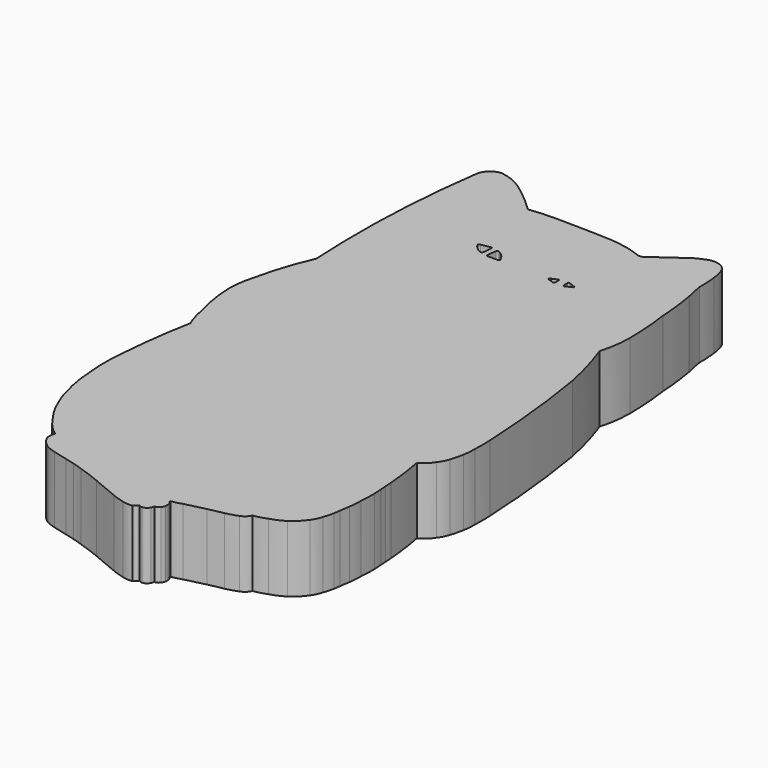
from build123d import *

# Parameters (mm, degrees)
F0_R     = 0.4870589974
F0_R_2   = 0.3474724492
F0_R_3   = 0.3665024193
F0_R_4   = 0.3542305884
F2_DEPTH = 15.24


# Not quite as in the source:
# - the program builds the solid bodies; features that only make, move or delete a surface that nothing else refers to are left out


with BuildPart() as f2:
    # F0 (on Top) → F2 (new body)
    with BuildSketch(Plane.XY):
        with BuildLine():
            ThreePointArc((-4.6574980952, 64.4998699427), (-8.9647320566, 64.5008636046), (-13.2575705647, 64.1490072012))
            ThreePointArc((-13.2575705647, 64.1490072012), (-16.5825370368, 67.1811284014), (-20.1327186078, 69.946154952))
            ThreePointArc((-20.1327186078, 69.946154952), (-22.7316970175, 71.3928848027), (-25.5997013301, 72.1817240119))
            ThreePointArc((-25.5997013301, 72.1817240119), (-27.9785809795, 71.1960010823), (-29.0786921978, 68.8678100705))
            ThreePointArc((-29.0786921978, 68.8678100705), (-31.0430656712, 47.2705474966), (-30.8605283499, 25.5849026144))
            ThreePointArc((-30.8605283499, 25.5849026144), (-33.274027732, 19.3250082515), (-35.0082106888, 12.843969278))
            ThreePointArc((-35.0082106888, 12.843969278), (-35.6586909212, 9.8700411989), (-35.8947664499, 6.8349726498))
            ThreePointArc((-35.8947664499, 6.8349726498), (-35.4181204016, 1.9087445697), (-34.3186743557, -2.9168261681))
            ThreePointArc((-34.3186743557, -2.9168261681), (-33.7425928924, -5.5247875256), (-32.8410901129, -8.0388728529))
            ThreePointArc((-32.8410901129, -8.0388728529), (-34.177182437, -16.2583737842), (-35.0319556892, -24.541772902))
            ThreePointArc((-35.0319556892, -24.541772902), (-35.3040614644, -29.3553117663), (-35.0319556892, -34.1688506305))
            ThreePointArc((-35.0319556892, -34.1688506305), (-34.5298956541, -38.6068361214), (-33.4818251431, -42.9484173656))
            ThreePointArc((-33.4818251431, -42.9484173656), (-33.0135473697, -44.5160756792), (-32.4171707034, -46.0396148264))
            ThreePointArc((-32.4171707034, -46.0396148264), (-31.9110692256, -47.2219894678), (-31.3906520605, -48.3981333673))
            ThreePointArc((-31.3906520605, -48.3981333673), (-30.5934071364, -49.8697175037), (-29.6822413802, -51.2736178935))
            ThreePointArc((-29.6822413802, -51.2736178935), (-28.7221089025, -52.6566027976), (-27.7248732746, -54.0130771697))
            ThreePointArc((-27.7248732746, -54.0130771697), (-26.4672846913, -55.3801105964), (-25.0454377383, -56.5753765404))
            Line((-25.0454377383, -56.5753765404), (-24.942945689, -56.6339418292))
            ThreePointArc((-24.942945689, -56.6339418292), (-25.1177355033, -57.0589329105), (-25.1918546855, -57.512447238))
            ThreePointArc((-25.1918546855, -57.512447238), (-25.1982887044, -58.3404447624), (-24.9355826527, -59.125687927))
            ThreePointArc((-24.9355826527, -59.125687927), (-24.0502846613, -60.3263263494), (-22.9040738195, -61.2810440361))
            ThreePointArc((-22.9040738195, -61.2810440361), (-21.8272966835, -61.7764366965), (-20.7001958042, -62.1431879699))
            ThreePointArc((-20.7001958042, -62.1431879699), (-19.0633016555, -62.5643833918), (-17.4251589924, -62.980696559))
            ThreePointArc((-17.4251589924, -62.980696559), (-16.3259212101, -63.2570568454), (-15.2335911989, -63.5595694184))
            ThreePointArc((-15.2335911989, -63.5595694184), (-14.0547489271, -63.8999797911), (-12.8942783922, -64.2985478044))
            ThreePointArc((-12.8942783922, -64.2985478044), (-10.3776553028, -65.1515690841), (-7.898459211, -66.1079287529))
            ThreePointArc((-7.898459211, -66.1079287529), (-4.843659707, -67.400231929), (-1.7793092411, -68.6697214842))
            ThreePointArc((-1.7793092411, -68.6697214842), (-0.4258068603, -69.1536416461), (0.953993469, -69.556504488))
            ThreePointArc((0.953993469, -69.556504488), (2.09089533, -69.7563797595), (3.2440575305, -69.7042942047))
            ThreePointArc((3.2440575305, -69.7042942047), (3.7517072509, -69.2953475436), (4.1341194883, -68.7674209476))
            ThreePointArc((4.1341194883, -68.7674209476), (4.4824361357, -69.0112523604), (4.9028098583, -69.0750032663))
            ThreePointArc((4.9028098583, -69.0750032663), (5.6978837565, -68.8446948411), (6.2388665974, -68.2181790471))
            ThreePointArc((6.2388665974, -68.2181790471), (6.3961650377, -67.8668892643), (6.4935988233, -67.4945265805))
            ThreePointArc((6.4935988233, -67.4945265805), (7.0853776684, -67.3748926573), (7.5344089419, -66.9713020325))
            ThreePointArc((7.5344089419, -66.9713020325), (7.7893950341, -66.5594064291), (7.9566510394, -66.1047622561))
            ThreePointArc((7.9566510394, -66.1047622561), (7.9580850948, -65.3933472028), (7.7242949046, -64.721442759))
            ThreePointArc((7.7242949046, -64.721442759), (7.6240357038, -64.5454642025), (7.4602863751, -64.4262731075))
            Line((7.4602863751, -64.4262731075), (7.4602863751, -64.1000345349))
            ThreePointArc((7.4602863751, -64.1000345349), (8.6957807292, -63.8684813987), (9.8980711773, -63.5016560555))
            ThreePointArc((9.8980711773, -63.5016560555), (12.1765605556, -62.956644983), (14.4535750151, -62.4055042863))
            ThreePointArc((14.4535750151, -62.4055042863), (16.1980956729, -62.0296921019), (17.9502312094, -61.6911537945))
            ThreePointArc((17.9502312094, -61.6911537945), (19.3508412218, -61.3167352774), (20.720468834, -60.8413219452))
            ThreePointArc((20.720468834, -60.8413219452), (21.7172842906, -60.2151089758), (22.3949253559, -59.2525154352))
            ThreePointArc((22.3949253559, -59.2525154352), (23.9413170616, -58.9427415638), (25.4360325634, -58.4396384656))
            ThreePointArc((25.4360325634, -58.4396384656), (27.0823885834, -57.8282787188), (28.6495089531, -57.0355728269))
            ThreePointArc((28.6495089531, -57.0355728269), (30.1858910448, -55.7262813708), (31.481307, -54.1781820357))
            ThreePointArc((31.481307, -54.1781820357), (32.1372272216, -53.052991053), (32.5707420707, -51.8248416483))
            ThreePointArc((32.5707420707, -51.8248416483), (32.9555178669, -50.6466711835), (33.2324020565, -49.4385845959))
            ThreePointArc((33.2324020565, -49.4385845959), (33.3537864539, -48.7541435906), (33.4239304066, -48.0625703931))
            ThreePointArc((33.4239304066, -48.0625703931), (33.5955437011, -46.9075690976), (33.7808765471, -45.7546897233))
            ThreePointArc((33.7808765471, -45.7546897233), (33.9514589063, -44.2393966213), (33.9985303581, -42.7152588964))
            ThreePointArc((33.9985303581, -42.7152588964), (34.1163088336, -40.8315734776), (34.118514508, -38.9442108572))
            ThreePointArc((34.118514508, -38.9442108572), (34.083978003, -37.9792527189), (33.9942798018, -37.0178520679))
            ThreePointArc((33.9942798018, -37.0178520679), (33.955975515, -36.2784612284), (33.8882356882, -35.5411842465))
            ThreePointArc((33.8882356882, -35.5411842465), (33.8712782201, -34.6642287786), (33.786136657, -33.7912514806))
            ThreePointArc((33.786136657, -33.7912514806), (33.3180795223, -29.3661557271), (32.5943753123, -24.9756202102))
            ThreePointArc((32.5943753123, -24.9756202102), (34.0489107492, -23.9527476363), (35.1713187993, -22.5735660642))
            ThreePointArc((35.1713187993, -22.5735660642), (35.9010770472, -21.4620836312), (36.4012233913, -20.2300958335))
            ThreePointArc((36.4012233913, -20.2300958335), (36.828967703, -18.7660485621), (37.1333099902, -17.2714665532))
            ThreePointArc((37.1333099902, -17.2714665532), (37.3389003532, -15.7697261697), (37.3675785959, -14.2542496324))
            ThreePointArc((37.3675785959, -14.2542496324), (37.4263640724, -12.1011873707), (37.3675785959, -9.9481251091))
            ThreePointArc((37.3675785959, -9.9481251091), (36.331409459, 3.6788193791), (34.4893857837, 17.2203928232))
            ThreePointArc((34.4893857837, 17.2203928232), (33.0120348597, 23.3170518073), (31.0925077647, 29.2892567813))
            ThreePointArc((31.0925077647, 29.2892567813), (31.8892450574, 32.9417140758), (32.1467109025, 36.6711840034))
            ThreePointArc((32.1467109025, 36.6711840034), (31.9281916192, 41.8984630944), (31.3738137484, 47.1008531749))
            ThreePointArc((31.3738137484, 47.1008531749), (30.9870656208, 51.5076967811), (30.3440932184, 55.8845028281))
            ThreePointArc((30.3440932184, 55.8845028281), (29.8980506559, 57.8596492724), (29.5387990773, 59.8524101079))
            ThreePointArc((29.5387990773, 59.8524101079), (29.5001644092, 62.03824233), (29.3045323342, 64.2156451941))
            ThreePointArc((29.3045323342, 64.2156451941), (29.0554228466, 65.8357987344), (28.5431630909, 67.3928931355))
            ThreePointArc((28.5431630909, 67.3928931355), (27.7313873665, 68.4152918791), (26.5811719, 69.0327733755))
            ThreePointArc((26.5811719, 69.0327733755), (25.4317978397, 69.2090389422), (24.2824237794, 69.0327733755))
            ThreePointArc((24.2824237794, 69.0327733755), (21.9444120738, 68.0189193625), (19.8459811509, 66.5729641914))
            ThreePointArc((19.8459811509, 66.5729641914), (17.3300117141, 64.7862316617), (14.8238698021, 62.985740602))
            ThreePointArc((14.8238698021, 62.985740602), (14.2064215735, 62.5788950359), (13.4768299758, 62.4586381018))
            ThreePointArc((13.4768299758, 62.4586381018), (11.0316395646, 63.3169292546), (8.4986444563, 63.8642460108))
            ThreePointArc((8.4986444563, 63.8642460108), (6.8510393358, 64.1197437557), (5.1896148361, 64.2595663667))
            ThreePointArc((5.1896148361, 64.2595663667), (0.2670117865, 64.4187870504), (-4.6574980952, 64.4998699427))
        make_face()
        with BuildLine():
            Line((-1.0718253907, -67.4767941236), (6.3647264615, -64.5711272955))
            ThreePointArc((6.3647264615, -64.5711272955), (6.9733703953, -65.3588843298), (6.8818381988, -66.3501615061))
            ThreePointArc((6.8818381988, -66.3501615061), (6.248455993, -66.5475154041), (5.7491185144, -66.9843032956))
            ThreePointArc((5.7491185144, -66.9843032956), (5.5498506128, -67.2328710451), (5.5274991319, -67.5506666303))
            ThreePointArc((5.5274991319, -67.5506666303), (5.4100983825, -67.8395088195), (5.1088854671, -67.9200291634))
            ThreePointArc((5.1088854671, -67.9200291634), (4.550994403, -67.8804673339), (4.0992875583, -67.5506666303))
            ThreePointArc((4.0992875583, -67.5506666303), (3.689928496, -67.5720046833), (3.3851813059, -67.8461566567))
            ThreePointArc((3.3851813059, -67.8461566567), (3.1917592991, -68.325763414), (2.8434458654, -68.7080100179))
            ThreePointArc((2.8434458654, -68.7080100179), (2.3263345356, -68.8067226844), (1.8092232058, -68.7080100179))
            ThreePointArc((1.8092232058, -68.7080100179), (0.3713994895, -68.2197332578), (-1.0718253907, -67.7476599813))
            ThreePointArc((-1.0718253907, -67.7476599813), (-1.1643120138, -67.6122270525), (-1.0718253907, -67.4767941236))
        make_face(mode=Mode.SUBTRACT)
        with BuildLine():
            ThreePointArc((-2.623158507, -65.6792148948), (-2.6954743039, -64.9004723873), (-2.5739099365, -64.1278848052))
            ThreePointArc((-2.5739099365, -64.1278848052), (-2.7480826507, -63.9151836223), (-3.017146606, -63.858769834))
            ThreePointArc((-3.017146606, -63.858769834), (-3.4181090068, -63.7899955014), (-3.7558770273, -63.5632500052))
            ThreePointArc((-3.7558770273, -63.5632500052), (-4.1021139481, -62.8983397037), (-3.7558770273, -62.2334294021))
            ThreePointArc((-3.7558770273, -62.2334294021), (-3.4445311977, -61.8172751284), (-3.4357607365, -61.2976178527))
            ThreePointArc((-3.4357607365, -61.2976178527), (-3.8185334208, -61.0520831854), (-4.2483638972, -60.9035976231))
            ThreePointArc((-4.2483638972, -60.9035976231), (-4.256998038, -60.2746639674), (-4.0759937838, -59.6722774208))
            ThreePointArc((-4.0759937838, -59.6722774208), (-2.988790696, -58.6144122793), (-1.6381832538, -57.923797518))
            ThreePointArc((-1.6381832538, -57.923797518), (1.1811274388, -56.897382154), (3.9022939745, -55.6335411966))
            ThreePointArc((3.9022939745, -55.6335411966), (5.981824211, -53.9429218927), (7.5466968119, -51.7671890557))
            ThreePointArc((7.5466968119, -51.7671890557), (8.3550122972, -52.4735297418), (9.368898347, -52.8261289001))
            ThreePointArc((9.368898347, -52.8261289001), (10.040849572, -52.6552470488), (9.9845072255, -51.9642010331))
            ThreePointArc((9.9845072255, -51.9642010331), (8.9657442091, -51.4896380021), (8.1130573526, -50.7575087249))
            ThreePointArc((8.1130573526, -50.7575087249), (7.7223088512, -49.166699086), (7.4235755019, -47.5560724735))
            ThreePointArc((7.4235755019, -47.5560724735), (7.2790449544, -44.2315042019), (7.4235755019, -40.9069359303))
            ThreePointArc((7.4235755019, -40.9069359303), (7.8475833512, -38.1104558628), (8.5316719487, -35.3659875691))
            ThreePointArc((8.5316719487, -35.3659875691), (9.546237916, -32.4876606134), (10.8463596553, -29.7265388072))
            ThreePointArc((10.8463596553, -29.7265388072), (12.7163248023, -26.7781756457), (15.0817465037, -24.2102202028))
            ThreePointArc((15.0817465037, -24.2102202028), (18.4017864047, -21.252419583), (22.2720559686, -19.0632957965))
            ThreePointArc((22.2720559686, -19.0632957965), (23.6866847639, -20.4435503048), (25.0792298466, -21.8460820615))
            ThreePointArc((25.0792298466, -21.8460820615), (28.1924648647, -24.0565281675), (31.6785536706, -25.6139263511))
            ThreePointArc((31.6785536706, -25.6139263511), (32.1205537257, -27.5065827192), (32.3926620185, -29.4310227036))
            ThreePointArc((32.3926620185, -29.4310227036), (32.7406981771, -31.9726512024), (32.9590179026, -34.5286913216))
            ThreePointArc((32.9590179026, -34.5286913216), (33.1425338772, -37.1117354068), (33.2052633166, -39.7005304694))
            ThreePointArc((33.2052633166, -39.7005304694), (33.1792019702, -43.1222482344), (32.7866487205, -46.521473676))
            ThreePointArc((32.7866487205, -46.521473676), (32.2374801563, -49.6606541109), (31.2106925994, -52.6775643229))
            ThreePointArc((31.2106925994, -52.6775643229), (29.6463762239, -54.7894621513), (27.5662895292, -56.3958361745))
            ThreePointArc((27.5662895292, -56.3958361745), (25.1040574774, -57.5429066445), (22.4444251508, -58.0949150026))
            ThreePointArc((22.4444251508, -58.0949150026), (22.1710291401, -57.487026745), (21.8780655414, -56.8883232772))
            ThreePointArc((21.8780655414, -56.8883232772), (21.2040875244, -56.5900957809), (20.8438429981, -57.2330653667))
            ThreePointArc((20.8438429981, -57.2330653667), (21.2474215961, -58.0165612606), (21.5086974204, -58.8582716882))
            ThreePointArc((21.5086974204, -58.8582716882), (20.6940197818, -59.6369824276), (19.661873579, -60.0894913077))
            Line((19.661873579, -60.0894913077), (7.3989494704, -63.0690380931))
            Line((7.3989494704, -63.0690380931), (2.3263345938, -64.7681206465))
            ThreePointArc((2.3263345938, -64.7681206465), (0.5926919978, -65.3977667437), (-1.0189079934, -66.2948265672))
            ThreePointArc((-1.0189079934, -66.2948265672), (-1.9152742777, -66.2326077196), (-2.623158507, -65.6792148948))
        make_face(mode=Mode.SUBTRACT)
        with Locations((-6.3439328223, 36.2661853433)):
            Circle(F0_R, mode=Mode.SUBTRACT)
        with Locations((-4.6601346694, 35.225212574)):
            Circle(F0_R_2, mode=Mode.SUBTRACT)
        with BuildLine():
            ThreePointArc((-24.7670784593, 67.2100633383), (-24.7422360081, 67.4660931138), (-24.5035272092, 67.5619393587))
            ThreePointArc((-24.5035272092, 67.5619393587), (-24.2630023675, 67.5067616438), (-24.0935590118, 67.3273578286))
            Line((-24.0935590118, 67.3273578286), (-20.2720686793, 63.7499317527))
            ThreePointArc((-20.2720686793, 63.7499317527), (-20.1529238407, 63.5519680773), (-20.1110094786, 63.3247494698))
            ThreePointArc((-20.1110094786, 63.3247494698), (-20.1793091244, 63.1254039906), (-20.3599203378, 63.0168542266))
            Line((-20.3599203378, 63.0168542266), (-23.2150536031, 61.3798877609))
            ThreePointArc((-23.2150536031, 61.3798877609), (-23.4814881607, 61.1666838735), (-23.8153655082, 61.0961914062))
            ThreePointArc((-23.8153655082, 61.0961914062), (-24.0717534356, 61.1512212134), (-24.1814088076, 61.3894201815))
            Line((-24.1814088076, 61.3894201815), (-24.7670784593, 67.2100633383))
        make_face(mode=Mode.SUBTRACT)
        with BuildLine():
            ThreePointArc((-9.2142317444, 48.5497191548), (-8.9722191607, 48.5070335326), (-8.8777504861, 48.2801683247))
            Line((-8.8777504861, 48.2801683247), (-9.1055221856, 46.1445078254))
            ThreePointArc((-9.1055221856, 46.1445078254), (-9.450986085, 45.9388162481), (-9.84578114, 46.0149161518))
            ThreePointArc((-9.84578114, 46.0149161518), (-10.8691429713, 46.7574912238), (-11.6886617616, 47.7203391492))
            ThreePointArc((-11.6886617616, 47.7203391492), (-11.6248552564, 48.0182618453), (-11.3677093759, 48.1816790998))
            Line((-11.3677093759, 48.1816790998), (-9.2142317444, 48.5497191548))
        make_face(mode=Mode.SUBTRACT)
        with BuildLine():
            ThreePointArc((0.0798076726, 36.0665917397), (-0.924263096, 37.2791040663), (-1.5656301985, 38.7168079615))
            ThreePointArc((-1.5656301985, 38.7168079615), (0.3771124535, 38.733779164), (2.2301948629, 38.1501503289))
            ThreePointArc((2.2301948629, 38.1501503289), (2.234031658, 38.0462048397), (2.1953706164, 37.9496403039))
            ThreePointArc((2.1953706164, 37.9496403039), (1.2064186028, 36.9307876648), (0.0798076726, 36.0665917397))
        make_face(mode=Mode.SUBTRACT)
        with BuildLine():
            ThreePointArc((-7.5725880452, 47.912247479), (-7.3780353415, 48.1541943288), (-7.067638915, 48.1476299465))
            ThreePointArc((-7.067638915, 48.1476299465), (-5.8641532243, 47.2968616284), (-5.030429922, 46.0815057158))
            ThreePointArc((-5.030429922, 46.0815057158), (-4.8961302642, 45.7175598685), (-5.1958444528, 45.4712584615))
            Line((-5.1958444528, 45.4712584615), (-7.4855275452, 45.4712584615))
            ThreePointArc((-7.4855275452, 45.4712584615), (-7.7517799665, 45.59444949), (-7.8685926273, 45.8635613322))
            Line((-7.8685926273, 45.8635613322), (-7.5725880452, 47.912247479))
        make_face(mode=Mode.SUBTRACT)
        with Locations((3.9052728098, 34.0376272798)):
            Circle(F0_R_3, mode=Mode.SUBTRACT)
        with Locations((6.3650822267, 34.961309284)):
            Circle(F0_R_4, mode=Mode.SUBTRACT)
        Polygon((5.4925759323, 45.4602651298), (8.4121963009, 46.7665418983), (8.5571417585, 44.3198606372), align=None, mode=Mode.SUBTRACT)
        Polygon((9.8616527393, 44.3198606372), (9.8616527393, 47.0153577626), (13.0711635575, 45.8542220294), align=None, mode=Mode.SUBTRACT)
        with BuildLine():
            ThreePointArc((19.9374128133, 59.918910265), (19.5176768801, 60.3374275402), (19.863538444, 60.8187951148))
            Line((19.863538444, 60.8187951148), (24.9115284532, 65.5284225941))
            ThreePointArc((24.9115284532, 65.5284225941), (25.740638025, 65.6767219123), (26.1427462101, 64.9366378784))
            Line((26.1427462101, 64.9366378784), (25.9457528591, 58.1311024725))
            ThreePointArc((25.9457528591, 58.1311024725), (25.9478496261, 57.8546128108), (25.6748851389, 57.8105524182))
            Line((25.6748851389, 57.8105524182), (19.9374128133, 59.918910265))
        make_face(mode=Mode.SUBTRACT)
        with BuildLine():
            ThreePointArc((-3.017146606, -63.858769834), (-2.7480826507, -63.9151836223), (-2.5739099365, -64.1278848052))
            ThreePointArc((-2.5739099365, -64.1278848052), (-2.6954743039, -64.9004723873), (-2.623158507, -65.6792148948))
            ThreePointArc((-2.623158507, -65.6792148948), (-1.9152742777, -66.2326077196), (-1.0189079934, -66.2948265672))
            ThreePointArc((-1.0189079934, -66.2948265672), (0.5926919978, -65.3977667437), (2.3263345938, -64.7681206465))
            Line((2.3263345938, -64.7681206465), (7.3989494704, -63.0690380931))
            Line((7.3989494704, -63.0690380931), (19.661873579, -60.0894913077))
            ThreePointArc((19.661873579, -60.0894913077), (20.6940197818, -59.6369824276), (21.5086974204, -58.8582716882))
            ThreePointArc((21.5086974204, -58.8582716882), (21.2474215961, -58.0165612606), (20.8438429981, -57.2330653667))
            ThreePointArc((20.8438429981, -57.2330653667), (21.2040875244, -56.5900957809), (21.8780655414, -56.8883232772))
            ThreePointArc((21.8780655414, -56.8883232772), (22.1710291401, -57.487026745), (22.4444251508, -58.0949150026))
            ThreePointArc((22.4444251508, -58.0949150026), (25.1040574774, -57.5429066445), (27.5662895292, -56.3958361745))
            ThreePointArc((27.5662895292, -56.3958361745), (29.6463762239, -54.7894621513), (31.2106925994, -52.6775643229))
            ThreePointArc((31.2106925994, -52.6775643229), (32.2374801563, -49.6606541109), (32.7866487205, -46.521473676))
            ThreePointArc((32.7866487205, -46.521473676), (33.1792019702, -43.1222482344), (33.2052633166, -39.7005304694))
            ThreePointArc((33.2052633166, -39.7005304694), (33.1425338772, -37.1117354068), (32.9590179026, -34.5286913216))
            ThreePointArc((32.9590179026, -34.5286913216), (32.7406981771, -31.9726512024), (32.3926620185, -29.4310227036))
            ThreePointArc((32.3926620185, -29.4310227036), (32.1205537257, -27.5065827192), (31.6785536706, -25.6139263511))
            ThreePointArc((31.6785536706, -25.6139263511), (28.1924648647, -24.0565281675), (25.0792298466, -21.8460820615))
            ThreePointArc((25.0792298466, -21.8460820615), (23.6866847639, -20.4435503048), (22.2720559686, -19.0632957965))
            ThreePointArc((22.2720559686, -19.0632957965), (18.4017864047, -21.252419583), (15.0817465037, -24.2102202028))
            ThreePointArc((15.0817465037, -24.2102202028), (12.7163248023, -26.7781756457), (10.8463596553, -29.7265388072))
            ThreePointArc((10.8463596553, -29.7265388072), (9.546237916, -32.4876606134), (8.5316719487, -35.3659875691))
            ThreePointArc((8.5316719487, -35.3659875691), (7.8475833512, -38.1104558628), (7.4235755019, -40.9069359303))
            ThreePointArc((7.4235755019, -40.9069359303), (7.2790449544, -44.2315042019), (7.4235755019, -47.5560724735))
            ThreePointArc((7.4235755019, -47.5560724735), (7.7223088512, -49.166699086), (8.1130573526, -50.7575087249))
            ThreePointArc((8.1130573526, -50.7575087249), (8.9657442091, -51.4896380021), (9.9845072255, -51.9642010331))
            ThreePointArc((9.9845072255, -51.9642010331), (10.040849572, -52.6552470488), (9.368898347, -52.8261289001))
            ThreePointArc((9.368898347, -52.8261289001), (8.3550122972, -52.4735297418), (7.5466968119, -51.7671890557))
            ThreePointArc((7.5466968119, -51.7671890557), (5.981824211, -53.9429218927), (3.9022939745, -55.6335411966))
            ThreePointArc((3.9022939745, -55.6335411966), (1.1811274388, -56.897382154), (-1.6381832538, -57.923797518))
            ThreePointArc((-1.6381832538, -57.923797518), (-2.988790696, -58.6144122793), (-4.0759937838, -59.6722774208))
            ThreePointArc((-4.0759937838, -59.6722774208), (-4.256998038, -60.2746639674), (-4.2483638972, -60.9035976231))
            ThreePointArc((-4.2483638972, -60.9035976231), (-3.8185334208, -61.0520831854), (-3.4357607365, -61.2976178527))
            ThreePointArc((-3.4357607365, -61.2976178527), (-3.4445311977, -61.8172751284), (-3.7558770273, -62.2334294021))
            ThreePointArc((-3.7558770273, -62.2334294021), (-4.1021139481, -62.8983397037), (-3.7558770273, -63.5632500052))
            ThreePointArc((-3.7558770273, -63.5632500052), (-3.4181090068, -63.7899955014), (-3.017146606, -63.858769834))
        make_face()
        with BuildLine():
            Line((24.9115284532, 65.5284225941), (19.863538444, 60.8187951148))
            ThreePointArc((19.863538444, 60.8187951148), (19.5176768801, 60.3374275402), (19.9374128133, 59.918910265))
            Line((19.9374128133, 59.918910265), (25.6748851389, 57.8105524182))
            ThreePointArc((25.6748851389, 57.8105524182), (25.9478496261, 57.8546128108), (25.9457528591, 58.1311024725))
            Line((25.9457528591, 58.1311024725), (26.1427462101, 64.9366378784))
            ThreePointArc((26.1427462101, 64.9366378784), (25.740638025, 65.6767219123), (24.9115284532, 65.5284225941))
        make_face()
        with BuildLine():
            Line((20.9922753274, 60.810495168), (24.698741734, 64.3975809216))
            ThreePointArc((24.698741734, 64.3975809216), (25.0690158468, 64.4878677154), (25.278525427, 64.1694962978))
            Line((25.278525427, 64.1694962978), (25.1128729433, 58.9858517051))
            ThreePointArc((25.1128729433, 58.9858517051), (24.8968366977, 58.6634817199), (24.5123840868, 58.7163046002))
            Line((24.5123840868, 58.7163046002), (20.9922753274, 59.918910265))
            ThreePointArc((20.9922753274, 59.918910265), (20.7188387044, 60.1168568588), (20.6032761511, 60.4340251692))
            Line((20.6032761511, 60.4340251692), (20.9922753274, 60.810495168))
        make_face(mode=Mode.SUBTRACT)
        with BuildLine():
            ThreePointArc((-24.0935590118, 67.3273578286), (-24.2630023675, 67.5067616438), (-24.5035272092, 67.5619393587))
            ThreePointArc((-24.5035272092, 67.5619393587), (-24.7422360081, 67.4660931138), (-24.7670784593, 67.2100633383))
            Line((-24.7670784593, 67.2100633383), (-24.1814088076, 61.3894201815))
            ThreePointArc((-24.1814088076, 61.3894201815), (-24.0717534356, 61.1512212134), (-23.8153655082, 61.0961914062))
            ThreePointArc((-23.8153655082, 61.0961914062), (-23.4814881607, 61.1666838735), (-23.2150536031, 61.3798877609))
            Line((-23.2150536031, 61.3798877609), (-20.3599203378, 63.0168542266))
            ThreePointArc((-20.3599203378, 63.0168542266), (-20.1793091244, 63.1254039906), (-20.1110094786, 63.3247494698))
            ThreePointArc((-20.1110094786, 63.3247494698), (-20.1529238407, 63.5519680773), (-20.2720686793, 63.7499317527))
            Line((-20.2720686793, 63.7499317527), (-24.0935590118, 67.3273578286))
        make_face()
        with BuildLine():
            ThreePointArc((6.8818381988, -66.3501615061), (6.9733703953, -65.3588843298), (6.3647264615, -64.5711272955))
            Line((6.3647264615, -64.5711272955), (-1.0718253907, -67.4767941236))
            ThreePointArc((-1.0718253907, -67.4767941236), (-1.1643120138, -67.6122270525), (-1.0718253907, -67.7476599813))
            ThreePointArc((-1.0718253907, -67.7476599813), (0.3713994895, -68.2197332578), (1.8092232058, -68.7080100179))
            ThreePointArc((1.8092232058, -68.7080100179), (2.3263345356, -68.8067226844), (2.8434458654, -68.7080100179))
            ThreePointArc((2.8434458654, -68.7080100179), (3.1917592991, -68.325763414), (3.3851813059, -67.8461566567))
            ThreePointArc((3.3851813059, -67.8461566567), (3.689928496, -67.5720046833), (4.0992875583, -67.5506666303))
            ThreePointArc((4.0992875583, -67.5506666303), (4.550994403, -67.8804673339), (5.1088854671, -67.9200291634))
            ThreePointArc((5.1088854671, -67.9200291634), (5.4100983825, -67.8395088195), (5.5274991319, -67.5506666303))
            ThreePointArc((5.5274991319, -67.5506666303), (5.5498506128, -67.2328710451), (5.7491185144, -66.9843032956))
            ThreePointArc((5.7491185144, -66.9843032956), (6.248455993, -66.5475154041), (6.8818381988, -66.3501615061))
        make_face()
        with BuildLine():
            ThreePointArc((25.278525427, 64.1694962978), (25.0690158468, 64.4878677154), (24.698741734, 64.3975809216))
            Line((24.698741734, 64.3975809216), (20.9922753274, 60.810495168))
            Line((20.9922753274, 60.810495168), (20.6032761511, 60.4340251692))
            ThreePointArc((20.6032761511, 60.4340251692), (20.7188387044, 60.1168568588), (20.9922753274, 59.918910265))
            Line((20.9922753274, 59.918910265), (24.5123840868, 58.7163046002))
            ThreePointArc((24.5123840868, 58.7163046002), (24.8968366977, 58.6634817199), (25.1128729433, 58.9858517051))
            Line((25.1128729433, 58.9858517051), (25.278525427, 64.1694962978))
        make_face()
        with BuildLine():
            ThreePointArc((2.2301948629, 38.1501503289), (0.3771124535, 38.733779164), (-1.5656301985, 38.7168079615))
            ThreePointArc((-1.5656301985, 38.7168079615), (-0.924263096, 37.2791040663), (0.0798076726, 36.0665917397))
            ThreePointArc((0.0798076726, 36.0665917397), (1.2064186028, 36.9307876648), (2.1953706164, 37.9496403039))
            ThreePointArc((2.1953706164, 37.9496403039), (2.234031658, 38.0462048397), (2.2301948629, 38.1501503289))
        make_face()
        Polygon((13.0711635575, 45.8542220294), (9.8616527393, 47.0153577626), (9.8616527393, 44.3198606372), align=None)
        with BuildLine():
            ThreePointArc((10.1400362328, 46.2667159736), (10.2771363797, 46.5388295828), (10.5748735368, 46.4740619063))
            Line((10.5748735368, 46.4740619063), (11.9311502203, 45.9349639714))
            ThreePointArc((11.9311502203, 45.9349639714), (12.0864630356, 45.8005599274), (11.9415037334, 45.6550493836))
            Line((11.9415037334, 45.6550493836), (10.6266392395, 44.9915416539))
            ThreePointArc((10.6266392395, 44.9915416539), (10.3185108103, 44.9638698643), (10.1607423276, 45.22998631))
            Line((10.1607423276, 45.22998631), (10.1400362328, 46.2667159736))
        make_face(mode=Mode.SUBTRACT)
        Polygon((8.5571417585, 44.3198606372), (8.4121963009, 46.7665418983), (5.4925759323, 45.4602651298), align=None)
        with BuildLine():
            ThreePointArc((7.8519657254, 46.2667159736), (8.0698650291, 46.328305012), (8.2350363955, 46.1734123528))
            Line((8.2350363955, 46.1734123528), (8.2764495164, 45.0952127576))
            ThreePointArc((8.2764495164, 45.0952127576), (8.0789712335, 44.8453884672), (7.7691394836, 44.9189692736))
            Line((7.7691394836, 44.9189692736), (6.6716936417, 45.2610887587))
            ThreePointArc((6.6716936417, 45.2610887587), (6.4157031332, 45.5392265392), (6.72345981, 45.7587204874))
            Line((6.72345981, 45.7587204874), (7.8519657254, 46.2667159736))
        make_face(mode=Mode.SUBTRACT)
        with Locations((-6.3439328223, 36.2661853433)):
            Circle(F0_R)
        with Locations((3.9052728098, 34.0376272798)):
            Circle(F0_R_3)
        with Locations((6.3650822267, 34.961309284)):
            Circle(F0_R_4)
        with Locations((-4.6601346694, 35.225212574)):
            Circle(F0_R_2)
    extrude(amount=F2_DEPTH)


solid = f2.part
